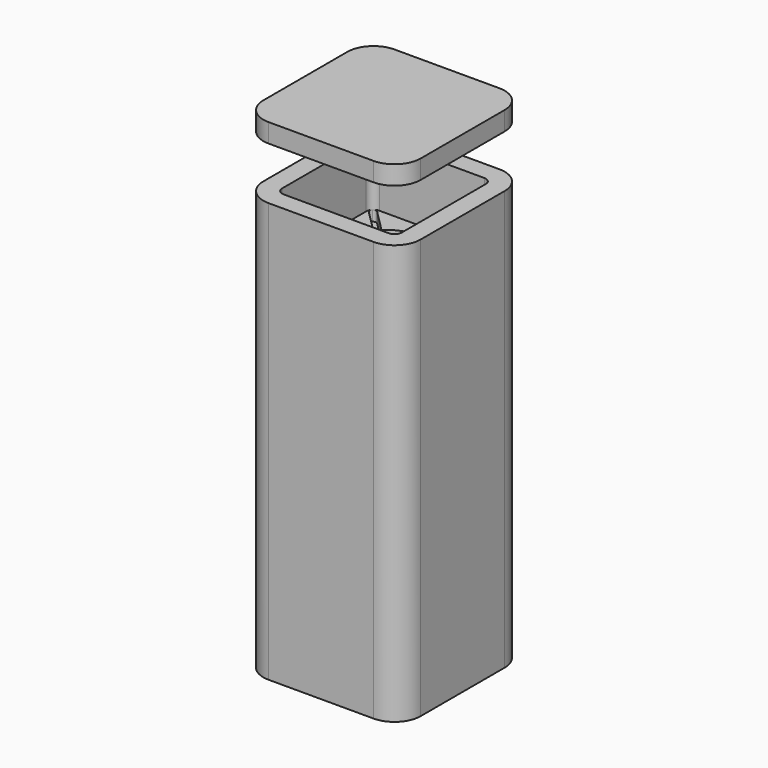
from build123d import *

# Parameters (mm, degrees)
F1_DEPTH  = 400
F2_T      = -18
F5_DEPTH  = 18
F7_R      = 45
F8_DEPTH  = 18
F10_DEPTH = 10
F12_DEPTH = 5
F13_R     = 3.09999


# Not quite as in the source:
# - a fillet or chamfer is up to 0.001 mm smaller than in the source, because OpenCascade refuses the exact size


with BuildPart() as f1:
    # F0 (on Top) → F1 (new body)
    with BuildSketch(Plane.XY):
        with BuildLine():
            ThreePointArc((-75, -50), (-67.6776695297, -67.6776695297), (-50, -75))
            Line((-50, -75), (50, -75))
            ThreePointArc((50, -75), (67.6776695297, -67.6776695297), (75, -50))
            Line((75, -50), (75, 50))
            ThreePointArc((75, 50), (67.6776695297, 67.6776695297), (50, 75))
            Line((50, 75), (-50, 75))
            ThreePointArc((-50, 75), (-67.6776695297, 67.6776695297), (-75, 50))
            Line((-75, 50), (-75, -50))
        make_face()
    extrude(amount=F1_DEPTH)

    # F2
    f2_openings = [f1.faces().sort_by_distance(p)[0] for p in [
        (0, 0, 400),
        (0, 0, 0),
    ]]
    offset(amount=F2_T, openings=f2_openings)

    # F7 (on offset) → F8 (join)
    with BuildSketch(Plane.XY.offset(340)):
        with BuildLine():
            Line((-57, 50), (-57, -50))
            ThreePointArc((-57, -50), (-54.9497474683, -54.9497474683), (-50, -57))
            Line((-50, -57), (50, -57))
            ThreePointArc((50, -57), (54.9497474683, -54.9497474683), (57, -50))
            Line((57, -50), (57, 50))
            ThreePointArc((57, 50), (54.9497474683, 54.9497474683), (50, 57))
            Line((50, 57), (-50, 57))
            ThreePointArc((-50, 57), (-54.9497474683, 54.9497474683), (-57, 50))
        make_face()
        Circle(F7_R, mode=Mode.SUBTRACT)
    extrude(amount=-F8_DEPTH)

    # F9 (on face) → F10 (cut)
    with BuildSketch(Plane.XY.offset(340)):
        with BuildLine():
            Line((54.9497474683, -50.5656854249), (33.9362430925, -29.5521810492))
            ThreePointArc((33.9362430925, -29.5521810492), (32.8975682992, -30.7042342357), (31.8198051534, -31.8198051534))
            ThreePointArc((31.8198051534, -31.8198051534), (30.7042342357, -32.8975682992), (29.5521810492, -33.9362430925))
            Line((29.5521810492, -33.9362430925), (50.5656854249, -54.9497474683))
            ThreePointArc((50.5656854249, -54.9497474683), (52.7577164727, -55.8577164466), (54.9497475052, -54.9497474314))
            ThreePointArc((54.9497475052, -54.9497474314), (55.8577164466, -52.7577164205), (54.9497474683, -50.5656854249))
        make_face()
        with BuildLine():
            ThreePointArc((-31.8198051534, -31.8198051534), (-32.8975682992, -30.7042342357), (-33.9362430925, -29.5521810492))
            Line((-33.9362430925, -29.5521810492), (-54.9497474683, -50.5656854249))
            ThreePointArc((-54.9497474683, -50.5656854249), (-55.8577164466, -52.7577164466), (-54.9497474683, -54.9497474683))
            ThreePointArc((-54.9497474683, -54.9497474683), (-52.7577164466, -55.8577164466), (-50.5656854249, -54.9497474683))
            Line((-50.5656854249, -54.9497474683), (-29.5521810492, -33.9362430925))
            ThreePointArc((-29.5521810492, -33.9362430925), (-30.7042342357, -32.8975682992), (-31.8198051534, -31.8198051534))
        make_face()
        with BuildLine():
            ThreePointArc((-33.9362430925, 29.5521810492), (-31.8198051534, 31.8198051534), (-29.5521810492, 33.9362430925))
            Line((-29.5521810492, 33.9362430925), (-50.5656854249, 54.9497474683))
            ThreePointArc((-50.5656854249, 54.9497474683), (-52.7577164628, 55.8577164466), (-54.9497474911, 54.9497474455))
            ThreePointArc((-54.9497474911, 54.9497474455), (-55.8577164466, 52.7577164305), (-54.9497474683, 50.5656854249))
            Line((-54.9497474683, 50.5656854249), (-33.9362430925, 29.5521810492))
        make_face()
        with BuildLine():
            ThreePointArc((29.5521810492, 33.9362430925), (31.8198051534, 31.8198051534), (33.9362430925, 29.5521810492))
            Line((33.9362430925, 29.5521810492), (54.9497474683, 50.5656854249))
            ThreePointArc((54.9497474683, 50.5656854249), (55.8577164466, 52.757716441), (54.9497474762, 54.9497474604))
            ThreePointArc((54.9497474762, 54.9497474604), (52.7577164522, 55.8577164466), (50.5656854249, 54.9497474683))
            Line((50.5656854249, 54.9497474683), (29.5521810492, 33.9362430925))
        make_face()
    extrude(amount=-F10_DEPTH, mode=Mode.SUBTRACT)


with BuildPart() as f5:
    # F4 (on offset) → F5 (new body)
    with BuildSketch(Plane.XY.offset(450)):
        with BuildLine():
            Line((-75, 50), (-75, -50))
            ThreePointArc((-75, -50), (-67.6776695297, -67.6776695297), (-50, -75))
            Line((-50, -75), (50, -75))
            ThreePointArc((50, -75), (67.6776695297, -67.6776695297), (75, -50))
            Line((75, -50), (75, 50))
            ThreePointArc((75, 50), (67.6776695297, 67.6776695297), (50, 75))
            Line((50, 75), (-50, 75))
            ThreePointArc((-50, 75), (-67.6776695297, 67.6776695297), (-75, 50))
        make_face()
    extrude(amount=F5_DEPTH)

    # F11 (on face) → F12 (cut)
    with BuildSketch(Plane(origin=(0, 0, 450), x_dir=(1, 0, 0), z_dir=(0, 0, -1))):
        Polygon((0, 4.3840620434), (-52.6087445203, 56.9928065636), (-56.9928065636, 52.6087445203), (-4.3840620434, 0), (-56.9928065636, -52.6087445203), (-52.6087445203, -56.9928065636), (0, -4.3840620434), (52.6087445203, -56.9928065636), (56.9928065636, -52.6087445203), (4.3840620434, 0), (56.9928065636, 52.6087445203), (52.6087445203, 56.9928065636), align=None)
    extrude(amount=-F12_DEPTH, mode=Mode.SUBTRACT)

    # F13 (radius 3.1 in the source; OpenCascade refuses exactly that, so slightly less here)
    f13_edges = [f5.edges().sort_by_distance(p)[0] for p in [
        (-52.608745, -56.992807, 452.5),
        (-56.992807, -52.608745, 452.5),
        (-56.992807, 52.608745, 452.5),
        (-52.608745, 56.992807, 452.5),
        (52.608745, 56.992807, 452.5),
        (56.992807, 52.608745, 452.5),
        (56.992807, -52.608745, 452.5),
        (52.608745, -56.992807, 452.5),
        (0, -4.384062, 452.5),
        (4.384062, 0, 452.5),
        (0, 4.384062, 452.5),
        (-4.384062, 0, 452.5),
    ]]
    fillet(f13_edges, radius=F13_R)


solid = Compound([f1.part, f5.part])
